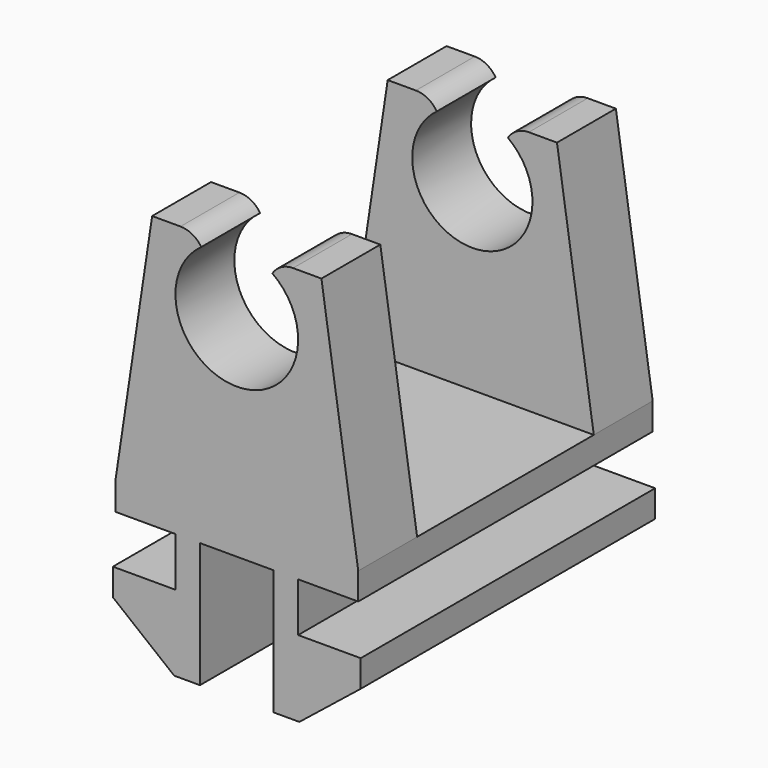
from build123d import *

# Parameters (mm, degrees)
F1_DEPTH     = 15
F3_DEPTH     = 25
F7_W         = 9.9
F7_H         = 3
F8_DEPTH     = 10
F10_DEPTH    = 3
F12_DEPTH    = 3
F13_T1_DEPTH = 7.2559990627
F13_T3_DEPTH = 7.2193706768


# Not quite as in the source:
# - a fillet or chamfer that OpenCascade refuses, or shapes differently, is made with other operations: its cross-section is extruded or revolved along the edge and cut away or added
# - a feature of the source that left no trace in its solid (it failed there, or was rolled back) is left out


with BuildPart() as f1:
    # F0 (on Front) → F1 (new body)
    with BuildSketch(Plane.XZ):
        Polygon((-2.5, 0.55), (-5.05, 0.55), (-5.05, -0.55), (-2.55, -2.55), (-1.5, -2.55), (-1.5, 2.55), (0, 2.55), (1.5, 2.55), (1.5, -2.55), (2.55, -2.55), (5.05, -0.55), (5.05, 0.55), (2.5, 0.55), (2.5, 2.55), (4.95, 2.55), (4.95, 3.65), (-4.95, 3.65), (-4.95, 2.55), (-2.5, 2.55), align=None)
    extrude(amount=F1_DEPTH)

    # F7 (on face) → F8 (join)
    with BuildSketch(Plane.XY.offset(3.65)):
        with Locations((0, -13.5)):
            Rectangle(F7_W, F7_H)
        with Locations((0, -1.5)):
            Rectangle(F7_W, F7_H)
    extrude(amount=F8_DEPTH)

    # F9 (on face) → F10 (cut, through all)
    with BuildSketch(Plane.XZ.offset(3)):
        with BuildLine():
            Line((-1.45, 13.65), (-1.45, 13.1748417658))
            ThreePointArc((-1.45, 13.1748417658), (0, 8.75), (1.45, 13.1748417658))
            Line((1.45, 13.1748417658), (1.45, 13.65))
            Line((1.45, 13.65), (-1.45, 13.65))
        make_face()
        Polygon((-4.95, 3.65), (-3.45, 13.65), (-4.95, 13.65), align=None)
        Polygon((4.95, 13.65), (3.45, 13.65), (4.95, 3.65), align=None)
    extrude(amount=-F10_DEPTH, mode=Mode.SUBTRACT)

    # F11 (on face) → F12 (cut, through all)
    with BuildSketch(Plane(origin=(0, -12, 0), x_dir=(-1, 0, 0), z_dir=(0, 1, 0))):
        with BuildLine():
            Line((-1.45, 13.65), (-1.45, 13.1865411854))
            ThreePointArc((-1.45, 13.1865411854), (0, 8.65), (1.45, 13.1865411854))
            Line((1.45, 13.1865411854), (1.45, 13.65))
            Line((1.45, 13.65), (-1.45, 13.65))
        make_face()
        Polygon((4.95, 13.65), (3.45, 13.65), (4.95, 3.65), align=None)
        Polygon((-4.95, 3.65), (-3.45, 13.65), (-4.95, 13.65), align=None)
    extrude(amount=-F12_DEPTH, mode=Mode.SUBTRACT)

    # F13: fillet of radius 1 on 4 edges, made by hand

    # F13_s2 → F13_t1 (cut)
    with BuildSketch(Plane.XZ.offset(-2.1279995313)):
        with BuildLine():
            ThreePointArc((1.45, 13.1748417658), (1.8137789296, 13.5231671563), (2.3011998125, 13.65))
            Line((2.3011998125, 13.65), (1.45, 13.65))
            Line((1.45, 13.65), (1.45, 13.1748417658))
        make_face()
        with BuildLine():
            ThreePointArc((-2.3011998125, 13.65), (-1.8137789296, 13.5231671563), (-1.45, 13.1748417658))
            Line((-1.45, 13.1748417658), (-1.45, 13.65))
            Line((-1.45, 13.65), (-2.3011998125, 13.65))
        make_face()
    extrude(amount=F13_T1_DEPTH, mode=Mode.SUBTRACT)

    # F13_s4 → F13_t3 (cut)
    with BuildSketch(Plane.XZ.offset(9.8903146616)):
        with BuildLine():
            ThreePointArc((1.45, 13.1865411854), (1.8124913279, 13.5265104636), (2.2938741354, 13.65))
            Line((2.2938741354, 13.65), (1.45, 13.65))
            Line((1.45, 13.65), (1.45, 13.1865411854))
        make_face()
        with BuildLine():
            ThreePointArc((-2.2938741354, 13.65), (-1.8124913279, 13.5265104636), (-1.45, 13.1865411854))
            Line((-1.45, 13.1865411854), (-1.45, 13.65))
            Line((-1.45, 13.65), (-2.2938741354, 13.65))
        make_face()
    extrude(amount=F13_T3_DEPTH, mode=Mode.SUBTRACT)


with BuildPart() as f3:
    # F2 (on face) → F3 (new body)
    with BuildSketch(Plane.XZ.offset(15)):
        with BuildLine():
            Line((-4.95, 3.65), (-4.0832418439, 3.65))
            Line((-4.0832418439, 3.65), (-0.75, 6.847274811))
            Line((-0.75, 6.847274811), (-0.75, 3.65))
            Line((-0.75, 3.65), (0.75, 3.65))
            Line((0.75, 3.65), (0.75, 6.828679691))
            Line((0.75, 6.828679691), (3.917720968, 3.65))
            Line((3.917720968, 3.65), (4.7647876878, 3.65))
            Line((4.7647876878, 3.65), (0.75, 7.6786768362))
            Line((0.75, 7.6786768362), (0.75, 7.9286768362))
            ThreePointArc((0.75, 7.9286768362), (0.6035533906, 8.2822302268), (0.25, 8.4286768362))
            Line((0.25, 8.4286768362), (-0.25, 8.4286768362))
            ThreePointArc((-0.25, 8.4286768362), (-0.6035533906, 8.2822302268), (-0.75, 7.9286768362))
            Line((-0.75, 7.9286768362), (-0.75, 7.6786768362))
            Line((-0.75, 7.6786768362), (-4.95, 3.65))
        make_face()
    extrude(amount=-F3_DEPTH)


solid = f1.part
